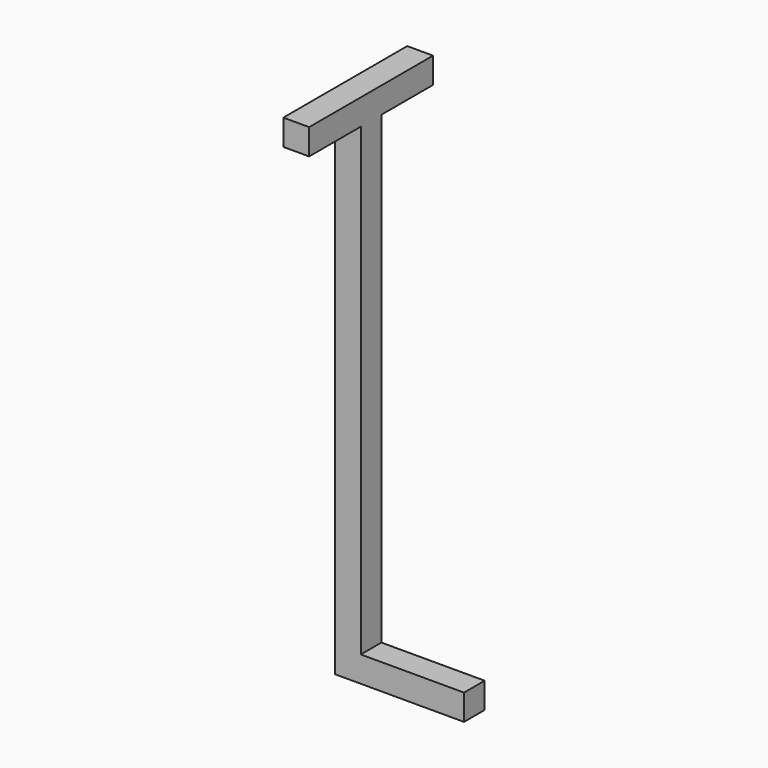
from build123d import *

# Parameters (mm, degrees)
F1_DEPTH = 25.4
F2_W     = 50.8
F2_H     = 50.8
F3_DEPTH = 127


# Not quite as in the source:
# - a feature of the source that left no trace in its solid (it failed there, or was rolled back) is left out
# - the program builds the solid bodies; features that only make, move or delete a surface that nothing else refers to are left out


with BuildPart() as f1:
    # F0 (on Front) → F1 (new body, symmetric)
    with BuildSketch(Plane.XZ):
        Polygon((0, -50.8), (0, 0), (-203.2, 0), (-203.2, 965.2), (-254, 965.2), (-254, -50.8), align=None)
    extrude(amount=F1_DEPTH, both=True)

    # F2 (on face) → F3 (join)
    with BuildSketch(Plane.XZ.offset(25.4)):
        with Locations((-228.6, 939.8)):
            Rectangle(F2_W, F2_H)
    extrude(amount=F3_DEPTH)

    # F4: F1 across plane


with BuildPart() as f1_1:
    add(f1.part)
    add(f1.part.mirror(Plane.XZ))


solid = f1_1.part
